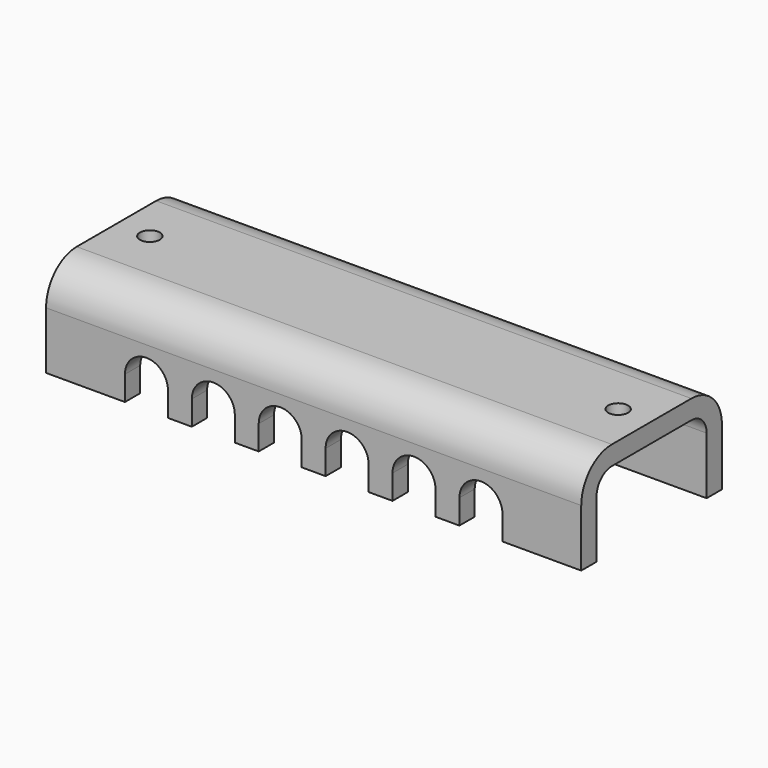
from build123d import *

# Parameters (mm, degrees)
F1_W     = 88.9
F1_H     = 29.21
F2_DEPTH = 3.175
F3_W     = 88.9
F3_H     = 3.175
F4_DEPTH = 12.7
F6_D     = 3.3
F8_DEPTH = 3.175
F9_R     = 6.35
F10_R    = 3.175


# Not quite as in the source:
# - a variable given as a bare number and used for a length is read in inches; the dataset says mm whatever the document's units were


with BuildPart() as f2:
    # F1 (on Top) → F2 (new body)
    with BuildSketch(Plane.XY):
        Rectangle(F1_W, F1_H)
    extrude(amount=F2_DEPTH)

    # F3 (on face) → F4 (join)
    with BuildSketch(Plane(origin=(0, 0, 0), x_dir=(1, 0, 0), z_dir=(0, 0, -1))):
        with Locations((0, 13.0175)):
            Rectangle(F3_W, F3_H)
        with Locations((0, -13.0175)):
            Rectangle(F3_W, F3_H)
    extrude(amount=F4_DEPTH)

    # F6 (through all)
    with Locations(Plane.XY.offset(3.175)):
        with Locations((-38.89375, 0), (38.89375, 0)):
            Hole(F6_D / 2)

    # F7 (on face) → F8 (cut)
    with BuildSketch(Plane.XZ.offset(14.605)):
        with BuildLine():
            Line((-31.353125, -8.636), (-24.209375, -8.636))
            ThreePointArc((-24.209375, -8.636), (-27.78125, -5.064125), (-31.353125, -8.636))
        make_face()
        with BuildLine():
            Line((-24.209375, -12.7), (-24.209375, -8.636))
            ThreePointArc((-24.209375, -8.636), (-27.78125, -12.207875), (-31.353125, -8.636))
            Line((-31.353125, -8.636), (-31.353125, -12.7))
            Line((-31.353125, -12.7), (-24.209375, -12.7))
        make_face()
        with BuildLine():
            ThreePointArc((-31.353125, -8.636), (-27.78125, -12.207875), (-24.209375, -8.636))
            Line((-24.209375, -8.636), (-31.353125, -8.636))
        make_face()
        with BuildLine():
            Line((-20.240625, -8.636), (-13.096875, -8.636))
            ThreePointArc((-13.096875, -8.636), (-16.66875, -5.064125), (-20.240625, -8.636))
        make_face()
        with BuildLine():
            Line((-13.096875, -12.7), (-13.096875, -8.636))
            ThreePointArc((-13.096875, -8.636), (-16.66875, -12.207875), (-20.240625, -8.636))
            Line((-20.240625, -8.636), (-20.240625, -12.7))
            Line((-20.240625, -12.7), (-13.096875, -12.7))
        make_face()
        with BuildLine():
            ThreePointArc((-20.240625, -8.636), (-16.66875, -12.207875), (-13.096875, -8.636))
            Line((-13.096875, -8.636), (-20.240625, -8.636))
        make_face()
        with BuildLine():
            Line((-9.128125, -8.636), (-1.984375, -8.636))
            ThreePointArc((-1.984375, -8.636), (-5.55625, -5.064125), (-9.128125, -8.636))
        make_face()
        with BuildLine():
            Line((-1.984375, -12.7), (-1.984375, -8.636))
            ThreePointArc((-1.984375, -8.636), (-5.55625, -12.207875), (-9.128125, -8.636))
            Line((-9.128125, -8.636), (-9.128125, -12.7))
            Line((-9.128125, -12.7), (-1.984375, -12.7))
        make_face()
        with BuildLine():
            ThreePointArc((-9.128125, -8.636), (-5.55625, -12.207875), (-1.984375, -8.636))
            Line((-1.984375, -8.636), (-9.128125, -8.636))
        make_face()
        with BuildLine():
            Line((1.984375, -8.636), (9.128125, -8.636))
            ThreePointArc((9.128125, -8.636), (5.55625, -5.064125), (1.984375, -8.636))
        make_face()
        with BuildLine():
            Line((9.128125, -12.7), (9.128125, -8.636))
            ThreePointArc((9.128125, -8.636), (5.55625, -12.207875), (1.984375, -8.636))
            Line((1.984375, -8.636), (1.984375, -12.7))
            Line((1.984375, -12.7), (9.128125, -12.7))
        make_face()
        with BuildLine():
            ThreePointArc((1.984375, -8.636), (5.55625, -12.207875), (9.128125, -8.636))
            Line((9.128125, -8.636), (1.984375, -8.636))
        make_face()
        with BuildLine():
            Line((13.096875, -8.636), (20.240625, -8.636))
            ThreePointArc((20.240625, -8.636), (16.66875, -5.064125), (13.096875, -8.636))
        make_face()
        with BuildLine():
            Line((20.240625, -12.7), (20.240625, -8.636))
            ThreePointArc((20.240625, -8.636), (16.66875, -12.207875), (13.096875, -8.636))
            Line((13.096875, -8.636), (13.096875, -12.7))
            Line((13.096875, -12.7), (20.240625, -12.7))
        make_face()
        with BuildLine():
            ThreePointArc((13.096875, -8.636), (16.66875, -12.207875), (20.240625, -8.636))
            Line((20.240625, -8.636), (13.096875, -8.636))
        make_face()
        with BuildLine():
            Line((24.209375, -8.636), (31.353125, -8.636))
            ThreePointArc((31.353125, -8.636), (27.78125, -5.064125), (24.209375, -8.636))
        make_face()
        with BuildLine():
            Line((31.353125, -12.7), (31.353125, -8.636))
            ThreePointArc((31.353125, -8.636), (27.78125, -12.207875), (24.209375, -8.636))
            Line((24.209375, -8.636), (24.209375, -12.7))
            Line((24.209375, -12.7), (31.353125, -12.7))
        make_face()
        with BuildLine():
            ThreePointArc((24.209375, -8.636), (27.78125, -12.207875), (31.353125, -8.636))
            Line((31.353125, -8.636), (24.209375, -8.636))
        make_face()
    extrude(amount=-F8_DEPTH, mode=Mode.SUBTRACT)

    # F9
    f9_edges = [f2.edges().sort_by_distance(p)[0] for p in [
        (0, -14.605, 3.175),
        (0, 14.605, 3.175),
    ]]
    fillet(f9_edges, radius=F9_R)

    # F10
    f10_edges = [f2.edges().sort_by_distance(p)[0] for p in [
        (0, 11.43, 0),
        (0, -11.43, 0),
    ]]
    fillet(f10_edges, radius=F10_R)


solid = f2.part
